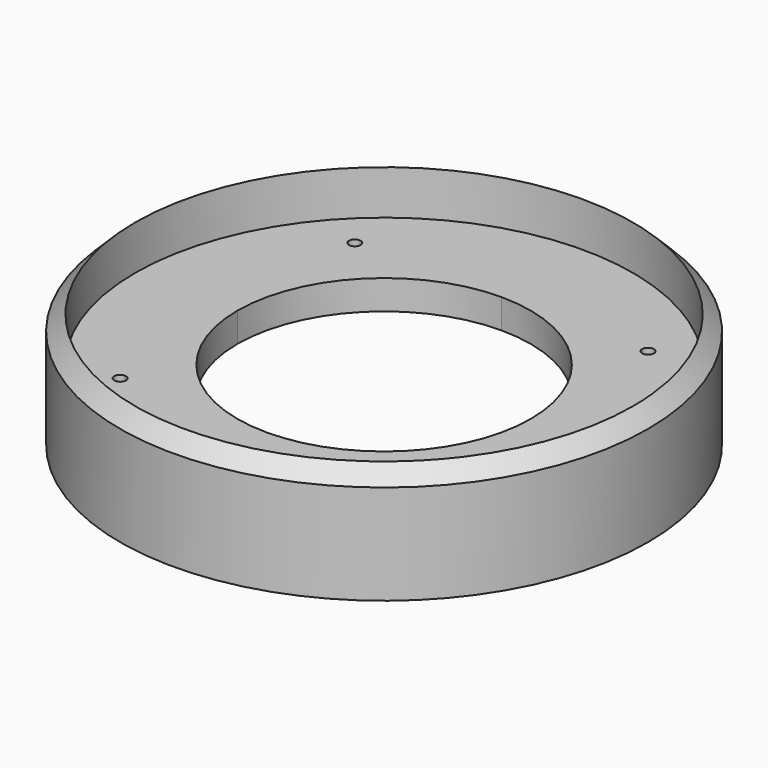
from build123d import *

# Parameters (mm, degrees)
F0_W     = 60
F0_H     = 60
F1_DEPTH = 5
F0_R     = 45
F2_DEPTH = 15
F4_DEPTH = 4
F5_DEPTH = 7


# Not quite as in the source:
# - a fillet or chamfer that OpenCascade refuses, or shapes differently, is made with other operations: its cross-section is extruded or revolved along the edge and cut away or added


with BuildPart() as f1:
    # F0 (on Top) → F1 (new body)
    with BuildSketch(Plane.XY):
        Rectangle(F0_W, F0_H)
        with BuildLine():
            Line((25, 24), (25, 0))
            Line((25, 0), (25, -24))
            ThreePointArc((25, -24), (25.7071067812, -24.2928932188), (26, -25))
            ThreePointArc((26, -25), (25, -26), (24, -25))
            Line((24, -25), (-5.83e-08, -25))
            Line((-5.83e-08, -25), (-24, -25))
            ThreePointArc((-24, -25), (-25.7071067812, -25.7071067812), (-25, -24))
            Line((-25, -24), (-25, 2.61e-08))
            Line((-25, 2.61e-08), (-25, 24))
            ThreePointArc((-25, 24), (-25.7071067812, 25.7071067812), (-24, 25))
            Line((-24, 25), (0, 25))
            Line((0, 25), (24, 25))
            ThreePointArc((24, 25), (25, 26), (26, 25))
            ThreePointArc((26, 25), (25.7071067812, 24.2928932188), (25, 24))
        make_face(mode=Mode.SUBTRACT)
        with BuildLine():
            ThreePointArc((0, 25), (17.6776695297, 17.6776695297), (25, 0))
            Line((25, 0), (25, 24))
            ThreePointArc((25, 24), (24.2928932188, 24.2928932188), (24, 25))
            Line((24, 25), (0, 25))
        make_face()
        with BuildLine():
            Line((30, 30), (30, -30))
            ThreePointArc((30, -30), (39.1968889463, -16.2358830044), (42.4264068712, 0))
            ThreePointArc((42.4264068712, 0), (39.1968889463, 16.2358830044), (30, 30))
        make_face()
        with BuildLine():
            ThreePointArc((-30, -30), (0, -42.4264068712), (30, -30))
            Line((30, -30), (-30, -30))
        make_face()
        with BuildLine():
            ThreePointArc((-30, 30), (-42.4264068712, 0), (-30, -30))
            Line((-30, -30), (-30, 30))
        make_face()
        with BuildLine():
            Line((-24, -25), (-5.83e-08, -25))
            ThreePointArc((-5.83e-08, -25), (-17.6776695595, -17.6776694998), (-25, 2.61e-08))
            Line((-25, 2.61e-08), (-25, -24))
            ThreePointArc((-25, -24), (-24.2928932188, -24.2928932188), (-24, -25))
        make_face()
        with BuildLine():
            Line((25, -24), (25, 0))
            ThreePointArc((25, 0), (17.677669509, -17.6776695503), (-5.83e-08, -25))
            Line((-5.83e-08, -25), (24, -25))
            ThreePointArc((24, -25), (24.2928932188, -24.2928932188), (25, -24))
        make_face()
        with BuildLine():
            ThreePointArc((-25, 2.61e-08), (-17.6776695204, 17.6776695389), (0, 25))
            Line((0, 25), (-24, 25))
            ThreePointArc((-24, 25), (-24.2928932188, 24.2928932188), (-25, 24))
            Line((-25, 24), (-25, 2.61e-08))
        make_face()
        with BuildLine():
            Line((-30, 30), (30, 30))
            ThreePointArc((30, 30), (0, 42.4264068712), (-30, 30))
        make_face()
    extrude(amount=F1_DEPTH)

    # F0 (on Top) → F2 (join)
    with BuildSketch(Plane.XY):
        Circle(F0_R)
        with BuildLine():
            ThreePointArc((42.4264068712, 0), (39.1968889463, -16.2358830044), (30, -30))
            ThreePointArc((30, -30), (0, -42.4264068712), (-30, -30))
            ThreePointArc((-30, -30), (-42.4264068712, 0), (-30, 30))
            ThreePointArc((-30, 30), (0, 42.4264068712), (30, 30))
            ThreePointArc((30, 30), (39.1968889463, 16.2358830044), (42.4264068712, 0))
        make_face(mode=Mode.SUBTRACT)
    extrude(amount=F2_DEPTH)

    # F3: chamfer of 5 on 1 edges, made by hand

    # F3_s1 → F3_t2 (revolve, cut)
    with BuildSketch(Plane.XZ):
        Polygon((40, 15), (45, 10), (45, 15), align=None)
    revolve(axis=Axis((0, 0, 15), (0, 0, 1)), mode=Mode.SUBTRACT)

    # F0 (on Top) → F4 (join)
    with BuildSketch(Plane.XY):
        Circle(F0_R)
        with BuildLine():
            ThreePointArc((42.4264068712, 0), (39.1968889463, -16.2358830044), (30, -30))
            ThreePointArc((30, -30), (0, -42.4264068712), (-30, -30))
            ThreePointArc((-30, -30), (-42.4264068712, 0), (-30, 30))
            ThreePointArc((-30, 30), (0, 42.4264068712), (30, 30))
            ThreePointArc((30, 30), (39.1968889463, 16.2358830044), (42.4264068712, 0))
        make_face(mode=Mode.SUBTRACT)
    extrude(amount=-F4_DEPTH)

    # F0 (on Top) → F5 (join)
    with BuildSketch(Plane.XY):
        Circle(F0_R)
        with BuildLine():
            ThreePointArc((42.4264068712, 0), (39.1968889463, -16.2358830044), (30, -30))
            ThreePointArc((30, -30), (0, -42.4264068712), (-30, -30))
            ThreePointArc((-30, -30), (-42.4264068712, 0), (-30, 30))
            ThreePointArc((-30, 30), (0, 42.4264068712), (30, 30))
            ThreePointArc((30, 30), (39.1968889463, 16.2358830044), (42.4264068712, 0))
        make_face(mode=Mode.SUBTRACT)
    extrude(amount=-F5_DEPTH)


solid = f1.part
